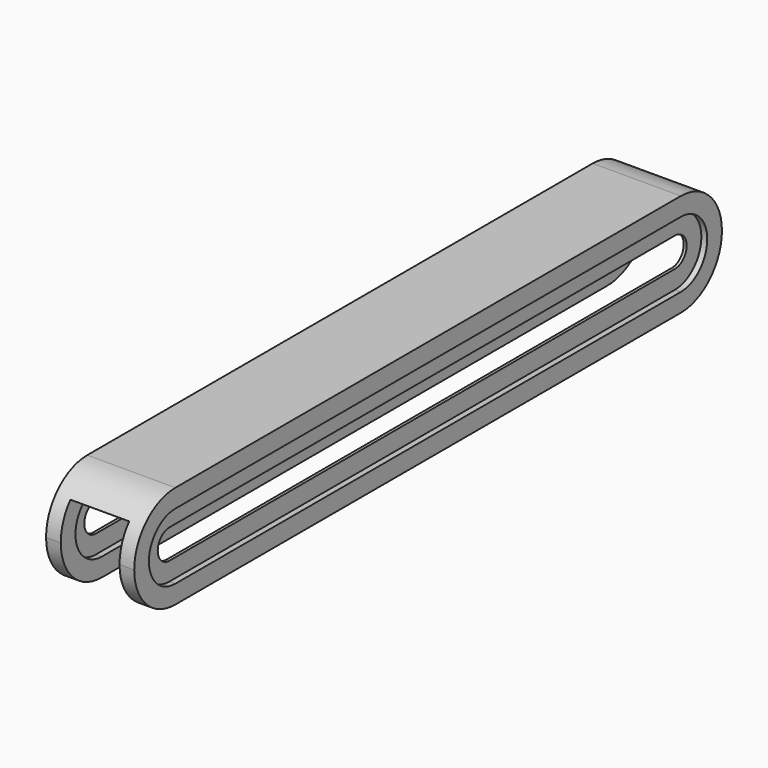
from build123d import *

# Parameters (mm, degrees)
F1_DEPTH      = 125
F1_DEPTH_BACK = 125
F6_DEPTH      = 5.001
F7_DEPTH      = 5.001
F8_DEPTH      = 2
F9_DEPTH      = 2
F10_DEPTH     = 2
F11_DEPTH     = 2
F12_T1_DEPTH  = 92.5
F12_T3_DEPTH  = 92.5
F12_T5_DEPTH  = 117.5


# Not quite as in the source:
# - a fillet or chamfer that OpenCascade refuses, or shapes differently, is made with other operations: its cross-section is extruded or revolved along the edge and cut away or added


with BuildPart() as f1:
    # F0 (on Front) → F1 (new body, two sides)
    with BuildSketch(Plane.XZ) as f1_sk:
        Polygon((15, -17.5), (15, 17.5), (-15, 17.5), (-15, -17.5), (-10, -17.5), (-10, 11.25), (10, 11.25), (10, -17.5), align=None)
    extrude(amount=F1_DEPTH)
    extrude(f1_sk.sketch, amount=-F1_DEPTH_BACK)

    # F2 (on face) → F6 (cut, through all)
    with BuildSketch(Plane(origin=(10, 0, 0), x_dir=(0, -1, 0), z_dir=(-1, 0, 0))):
        with BuildLine():
            Line((-107.5, -5), (107.5, -5))
            ThreePointArc((107.5, -5), (112.5, 0), (107.5, 5))
            Line((107.5, 5), (-107.5, 5))
            ThreePointArc((-107.5, 5), (-112.5, 0), (-107.5, -5))
        make_face()
    extrude(amount=-F6_DEPTH, mode=Mode.SUBTRACT)

    # F4 (on face) → F7 (cut, through all)
    with BuildSketch(Plane.YZ.offset(-10)):
        with BuildLine():
            Line((107.5, 5), (-107.5, 5))
            ThreePointArc((-107.5, 5), (-112.5, 0), (-107.5, -5))
            Line((-107.5, -5), (107.5, -5))
            ThreePointArc((107.5, -5), (112.5, 0), (107.5, 5))
        make_face()
    extrude(amount=-F7_DEPTH, mode=Mode.SUBTRACT)

    # F2 (on face) → F8 (cut)
    with BuildSketch(Plane(origin=(10, 0, 0), x_dir=(0, -1, 0), z_dir=(-1, 0, 0))):
        with BuildLine():
            Line((-107.5, -11.25), (107.5, -11.25))
            ThreePointArc((107.5, -11.25), (118.75, 0), (107.5, 11.25))
            Line((107.5, 11.25), (-107.5, 11.25))
            ThreePointArc((-107.5, 11.25), (-118.75, 0), (-107.5, -11.25))
        make_face()
        with BuildLine():
            ThreePointArc((107.5, 5), (112.5, 0), (107.5, -5))
            Line((107.5, -5), (-107.5, -5))
            ThreePointArc((-107.5, -5), (-112.5, 0), (-107.5, 5))
            Line((-107.5, 5), (107.5, 5))
        make_face(mode=Mode.SUBTRACT)
    extrude(amount=-F8_DEPTH, mode=Mode.SUBTRACT)

    # F3 (on face) → F9 (cut)
    with BuildSketch(Plane.YZ.offset(15)):
        with BuildLine():
            ThreePointArc((-107.5, 11.25), (-118.75, 0), (-107.5, -11.25))
            Line((-107.5, -11.25), (107.5, -11.25))
            ThreePointArc((107.5, -11.25), (118.75, 0), (107.5, 11.25))
            Line((107.5, 11.25), (-107.5, 11.25))
        make_face()
        with BuildLine():
            ThreePointArc((-107.5, -5), (-112.5, 0), (-107.5, 5))
            Line((-107.5, 5), (107.5, 5))
            ThreePointArc((107.5, 5), (112.5, 0), (107.5, -5))
            Line((107.5, -5), (-107.5, -5))
        make_face(mode=Mode.SUBTRACT)
    extrude(amount=-F9_DEPTH, mode=Mode.SUBTRACT)

    # F5 (on face) → F10 (cut)
    with BuildSketch(Plane(origin=(-15, 0, 0), x_dir=(0, -1, 0), z_dir=(-1, 0, 0))):
        with BuildLine():
            Line((107.5, 11.25), (-107.5, 11.25))
            ThreePointArc((-107.5, 11.25), (-118.75, 0), (-107.5, -11.25))
            Line((-107.5, -11.25), (107.5, -11.25))
            ThreePointArc((107.5, -11.25), (118.75, 0), (107.5, 11.25))
        make_face()
        with BuildLine():
            ThreePointArc((-107.5, -5), (-112.5, 0), (-107.5, 5))
            Line((-107.5, 5), (107.5, 5))
            ThreePointArc((107.5, 5), (112.5, 0), (107.5, -5))
            Line((107.5, -5), (-107.5, -5))
        make_face(mode=Mode.SUBTRACT)
    extrude(amount=-F10_DEPTH, mode=Mode.SUBTRACT)

    # F4 (on face) → F11 (cut)
    with BuildSketch(Plane.YZ.offset(-10)):
        with BuildLine():
            Line((107.5, 11.25), (-107.5, 11.25))
            ThreePointArc((-107.5, 11.25), (-118.75, 0), (-107.5, -11.25))
            Line((-107.5, -11.25), (107.5, -11.25))
            ThreePointArc((107.5, -11.25), (118.75, 0), (107.5, 11.25))
        make_face()
        with BuildLine():
            ThreePointArc((-107.5, -5), (-112.5, 0), (-107.5, 5))
            Line((-107.5, 5), (107.5, 5))
            ThreePointArc((107.5, 5), (112.5, 0), (107.5, -5))
            Line((107.5, -5), (-107.5, -5))
        make_face(mode=Mode.SUBTRACT)
    extrude(amount=-F11_DEPTH, mode=Mode.SUBTRACT)

    # F12: fillet of radius 17.5 on 6 edges, made by hand

    # F12_s2 → F12_t1 (cut)
    with BuildSketch(Plane.YZ.offset(-58.75)):
        with BuildLine():
            ThreePointArc((125, 0), (119.8743686708, -12.3743686708), (107.5, -17.5))
            Line((107.5, -17.5), (125, -17.5))
            Line((125, -17.5), (125, 0))
        make_face()
        with BuildLine():
            ThreePointArc((-125, 0), (-119.8743686708, -12.3743686708), (-107.5, -17.5))
            Line((-107.5, -17.5), (-125, -17.5))
            Line((-125, -17.5), (-125, 0))
        make_face()
    extrude(amount=F12_T1_DEPTH, mode=Mode.SUBTRACT)

    # F12_s4 → F12_t3 (cut)
    with BuildSketch(Plane.YZ.offset(-33.75)):
        with BuildLine():
            ThreePointArc((107.5, -17.5), (119.8743686708, -12.3743686708), (125, 0))
            Line((125, 0), (125, -17.5))
            Line((125, -17.5), (107.5, -17.5))
        make_face()
        with BuildLine():
            ThreePointArc((-107.5, -17.5), (-119.8743686708, -12.3743686708), (-125, 0))
            Line((-125, 0), (-125, -17.5))
            Line((-125, -17.5), (-107.5, -17.5))
        make_face()
    extrude(amount=F12_T3_DEPTH, mode=Mode.SUBTRACT)

    # F12_s6 → F12_t5 (cut)
    with BuildSketch(Plane.YZ.offset(-58.75)):
        with BuildLine():
            ThreePointArc((125, 0), (119.8743686708, 12.3743686708), (107.5, 17.5))
            Line((107.5, 17.5), (125, 17.5))
            Line((125, 17.5), (125, 0))
        make_face()
        with BuildLine():
            ThreePointArc((-125, 0), (-119.8743686708, 12.3743686708), (-107.5, 17.5))
            Line((-107.5, 17.5), (-125, 17.5))
            Line((-125, 17.5), (-125, 0))
        make_face()
    extrude(amount=F12_T5_DEPTH, mode=Mode.SUBTRACT)


solid = f1.part
